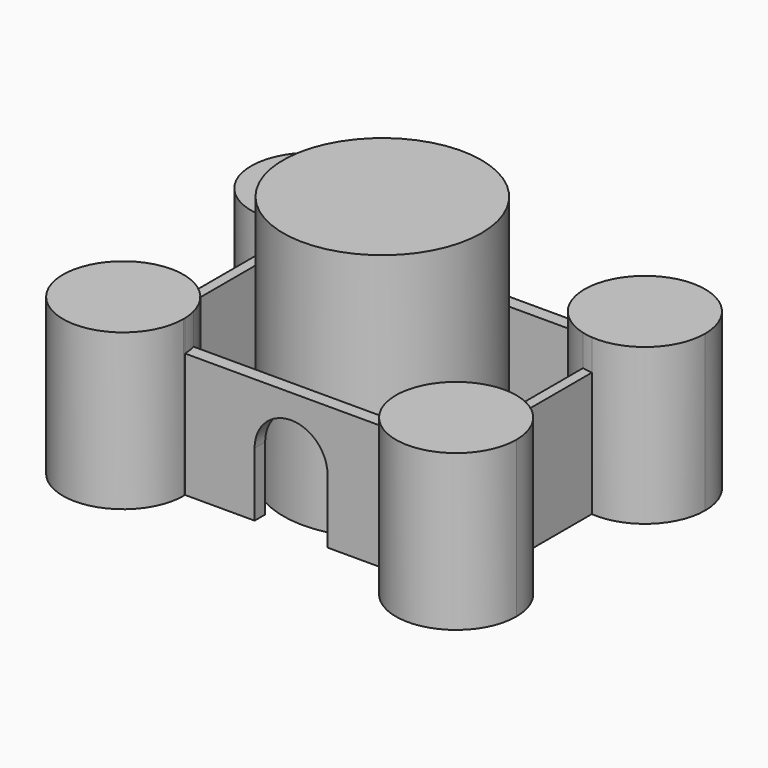
from build123d import *

# Parameters (mm, degrees)
F1_DEPTH = 25.4
F2_DEPTH = 31.75
F0_R     = 20.2081200016
F3_DEPTH = 50.8
F5_DEPTH = 25.4


with BuildPart() as f1:
    # F0 (on Top) → F1 (new body)
    with BuildSketch(Plane.XY):
        with BuildLine():
            Line((22.2428232494, 23.7755812705), (-21.2090998951, 23.7755812705))
            ThreePointArc((-21.2090998951, 23.7755812705), (-21.2837375348, 22.4235288232), (-21.5067434167, 21.0879072547))
            Line((-21.5067434167, 21.0879072547), (22.5404667711, 21.0879072547))
            ThreePointArc((22.5404667711, 21.0879072547), (22.3174608892, 22.4235288232), (22.2428232494, 23.7755812705))
        make_face()
    extrude(amount=F1_DEPTH)


with BuildPart() as f1b:
    # F0 (on Top) → F1, piece 2 (new body)
    with BuildSketch(Plane.XY):
        with BuildLine():
            Line((33.4925577044, -11.2923389787), (33.4925577044, 11.5356976198))
            ThreePointArc((33.4925577044, 11.5356976198), (32.4511353861, 11.6686780251), (31.4248725772, 11.8901026859))
            Line((31.4248725772, 11.8901026859), (31.4248725772, -11.5385687696))
            ThreePointArc((31.4248725772, -11.5385687696), (32.4534881194, -11.3715605888), (33.4925577044, -11.2923389787))
        make_face()
    extrude(amount=F1_DEPTH)


with BuildPart() as f1c:
    # F0 (on Top) → F1, piece 3 (new body)
    with BuildSketch(Plane.XY):
        with BuildLine():
            Line((21.8756893355, -21.0879072547), (-21.6070149652, -21.0879072547))
            ThreePointArc((-21.6070149652, -21.0879072547), (-21.3370268115, -22.4209057163), (-21.2160613421, -23.7755812705))
            Line((-21.2160613421, -23.7755812705), (21.6242800548, -23.7755812705))
            ThreePointArc((21.6242800548, -23.7755812705), (21.675930241, -22.4248170917), (21.8756893355, -21.0879072547))
        make_face()
    extrude(amount=F1_DEPTH)

    # F4 (on face) → F5 (cut)
    with BuildSketch(Plane.XZ.offset(23.7755812705)):
        with BuildLine():
            Line((-7.0293024182, 13.0248842761), (-7.0293024182, 0))
            Line((-7.0293024182, 0), (7.8562796116, 0))
            Line((7.8562796116, 0), (7.8562796116, 13.0248842761))
            ThreePointArc((7.8562796116, 13.0248842761), (0.4134885967, 20.467675291), (-7.0293024182, 13.0248842761))
        make_face()
    extrude(amount=-F5_DEPTH, mode=Mode.SUBTRACT)


with BuildPart() as f1d:
    # F0 (on Top) → F1, piece 4 (new body)
    with BuildSketch(Plane.XY):
        with BuildLine():
            ThreePointArc((-31.4248725772, 11.6674016398), (-32.4550071966, 11.5360214459), (-33.4925577044, 11.4921234611))
            Line((-33.4925577044, 11.4921234611), (-33.4925577044, -11.9056120578))
            ThreePointArc((-33.4925577044, -11.9056120578), (-32.4550071966, -11.9495100426), (-31.4248725772, -12.0808902364))
            Line((-31.4248725772, -12.0808902364), (-31.4248725772, 11.6674016398))
        make_face()
    extrude(amount=F1_DEPTH)


with BuildPart() as f2:
    # F0 (on Top) → F2 (new body)
    with BuildSketch(Plane.XY):
        with BuildLine():
            ThreePointArc((-21.5067434167, 21.0879072547), (-21.2837375348, 22.4235288232), (-21.2090998951, 23.7755812705))
            ThreePointArc((-21.2090998951, 23.7755812705), (-42.1782740179, 32.4612975839), (-33.4925577044, 11.4921234611))
            ThreePointArc((-33.4925577044, 11.4921234611), (-32.4550071966, 11.5360214459), (-31.4248725772, 11.6674016398))
            ThreePointArc((-31.4248725772, 11.6674016398), (-25.0331432471, 14.8693114119), (-21.5067434167, 21.0879072547))
        make_face()
    extrude(amount=F2_DEPTH)


with BuildPart() as f2b:
    # F0 (on Top) → F2, piece 2 (new body)
    with BuildSketch(Plane.XY):
        with BuildLine():
            ThreePointArc((-31.4248725772, -12.0808902364), (-32.4550071966, -11.9495100426), (-33.4925577044, -11.9056120578))
            ThreePointArc((-33.4925577044, -11.9056120578), (-42.1782740179, -32.8747861806), (-21.2090998951, -24.1890698671))
            ThreePointArc((-21.2090998951, -24.1890698671), (-21.2108403801, -23.9822962703), (-21.2160613421, -23.7755812705))
            ThreePointArc((-21.2160613421, -23.7755812705), (-21.3370268115, -22.4209057163), (-21.6070149652, -21.0879072547))
            ThreePointArc((-21.6070149652, -21.0879072547), (-25.1886591703, -15.137627723), (-31.4248725772, -12.0808902364))
        make_face()
    extrude(amount=F2_DEPTH)


with BuildPart() as f2c:
    # F0 (on Top) → F2, piece 3 (new body)
    with BuildSketch(Plane.XY):
        with BuildLine():
            ThreePointArc((46.8097388682, 23.7755812705), (34.5262810588, 36.0590390798), (22.2428232494, 23.7755812705))
            ThreePointArc((22.2428232494, 23.7755812705), (22.3174608892, 22.4235288232), (22.5404667711, 21.0879072547))
            ThreePointArc((22.5404667711, 21.0879072547), (25.6913518036, 15.2416864498), (31.4248725772, 11.8901026859))
            ThreePointArc((31.4248725772, 11.8901026859), (32.4511353861, 11.6686780251), (33.4925577044, 11.5356976198))
            ThreePointArc((33.4925577044, 11.5356976198), (42.8384901077, 14.7317703214), (46.8097388682, 23.7755812705))
        make_face()
    extrude(amount=F2_DEPTH)


with BuildPart() as f2d:
    # F0 (on Top) → F2, piece 4 (new body)
    with BuildSketch(Plane.XY):
        with BuildLine():
            ThreePointArc((46.1894556817, -23.5688369721), (42.4442898823, -14.7381571961), (33.4925577044, -11.2923389787))
            ThreePointArc((33.4925577044, -11.2923389787), (32.4534881194, -11.3715605888), (31.4248725772, -11.5385687696))
            ThreePointArc((31.4248725772, -11.5385687696), (25.2202109569, -14.8831912613), (21.8756893355, -21.0879072547))
            ThreePointArc((21.8756893355, -21.0879072547), (21.675930241, -22.4248170917), (21.6242800548, -23.7755812705))
            ThreePointArc((21.6242800548, -23.7755812705), (34.0093736825, -35.8518597758), (46.1894556817, -23.5688369721))
        make_face()
    extrude(amount=F2_DEPTH)


with BuildPart() as f3:
    # F0 (on Top) → F3 (new body)
    with BuildSketch(Plane.XY):
        Circle(F0_R)
    extrude(amount=F3_DEPTH)


solid = Compound([f1.part, f1b.part, f1c.part, f1d.part, f2.part, f2b.part, f2c.part, f2d.part, f3.part])
